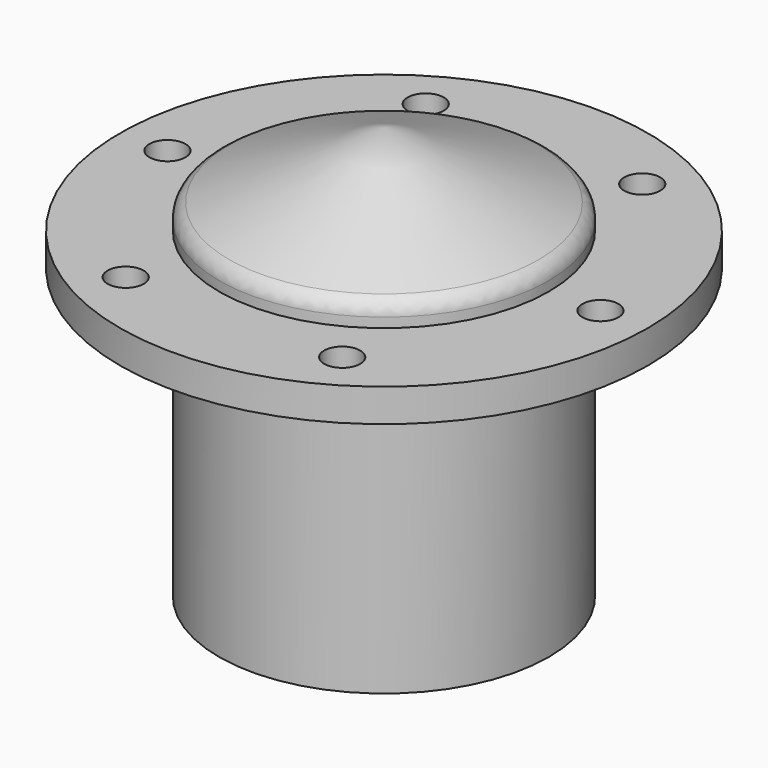
from build123d import *

# Parameters (mm, degrees)
F3_D            = 5.5626
F3_COPIES_COUNT = 6
F4_R            = 2.54
F5_T            = 4.572


# Not quite as in the source:
# - a pattern or mirror of a feature is missing from the dataset's text; its kind, count and spacing are read off the source's solid
# - a shell that OpenCascade refuses in one call is made with other operations: the cavity is built on its own and cut out


with BuildPart() as f2:
    # F1 (on Front) → F2 (revolve)
    with BuildSketch(Plane.XZ):
        Polygon((25.4, 8.255), (0, 19.05), (0, -44.45), (25.4, -44.45), (25.4, 0), (40.64, 0), (40.64, 5.08), (25.4, 5.08), align=None)
    revolve(axis=Axis((0, 0, -12.7), (0, 0, 1)))

    # F3 (through all)
    with Locations(Plane(origin=(0, 0, 0), x_dir=(1, 0, 0), z_dir=(0, 0, -1))):
        with Locations((33.3375, 0)):
            f3 = Hole(F3_D / 2)

    # F3_copies: F3 ×6 about axis
    f3_copies_axis = Axis((0, 0, 0), (0, 0, 1))
    for i in range(1, F3_COPIES_COUNT):
        add(f3.rotate(f3_copies_axis, i * 360 / F3_COPIES_COUNT), mode=Mode.SUBTRACT)

    # F4
    f4_edges = [f2.edges().sort_by_distance(p)[0] for p in [
        (-25.4, 0, 8.255),
    ]]
    fillet(f4_edges, radius=F4_R)

    # F5: shell of thickness 4.572, made by hand


with BuildPart() as f5_core1:
    # F5_t2: copy of F2
    add(f2.part)

    # the walls: a layer under each face that stays
    f5_faces = [f5_core1.faces().sort_by_distance(p)[0] for p in [
        (-25.4, 0, 5.8273115729),
        (-24.9783818064, 0, 7.9760718686),
        (-27.0933333333, -27.0933333333, 5.08),
        (-11.9267486132, 0, 13.9811318394),
        (-40.64, 0, 2.54),
        (-15.2781, -26.4624454431, 2.54),
        (15.2781, -26.4624454431, 2.54),
        (30.5562, 0, 2.54),
        (-30.5562, 0, 2.54),
        (-15.2781, 26.4624454431, 2.54),
        (15.2781, 26.4624454431, 2.54),
        (27.0933333333, -27.0933333333, 0),
        (-25.4, 0, -22.225),
    ]]
    thicken(f5_faces, amount=-F5_T, mode=Mode.SUBTRACT)

    # F5_s3 → F5_t4 (revolve, cut)
    with BuildSketch(Plane.XZ):
        Polygon((25.44572, 5.12572), (20.828, 5.08), (20.828, 0.508), (25.4, 0.508), align=None)
    revolve(axis=Axis((0, 0, 5.08), (0, 0, 1)), mode=Mode.SUBTRACT)

    # F5_s5 → F5_t6 (revolve, cut)
    with BuildSketch(Plane.XZ):
        Polygon((25.44572, -0.04572), (25.4, 4.572), (20.828, 4.572), (20.828, 0), align=None)
    revolve(axis=Axis((0, 0, 0), (0, 0, 1)), mode=Mode.SUBTRACT)


with BuildPart() as f2_1:
    add(f2.part)

    # what is left inside the walls is the cavity
    f5_cavity = [f5_core1.part.solids().sort_by_distance(p)[0] for p in [
        (-20.78228, 0, -29.633333),
    ]]
    add(f5_cavity, mode=Mode.SUBTRACT)


solid = f2_1.part
